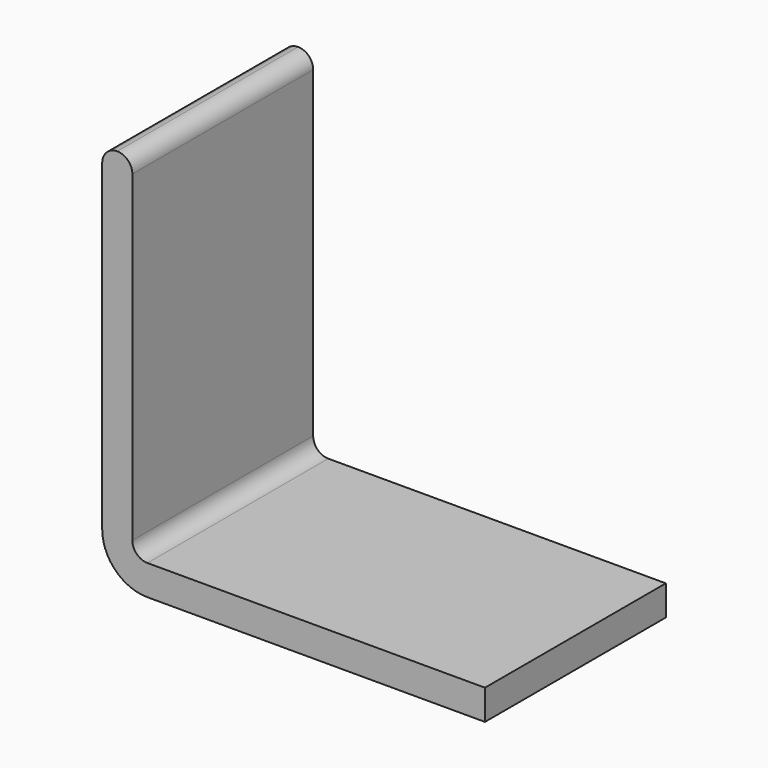
from build123d import *

# Parameters (mm, degrees)
F1_DEPTH = 7.5
F2_R     = 0.99999


# Not quite as in the source:
# - a fillet or chamfer is up to 0.001 mm smaller than in the source, because OpenCascade refuses the exact size


with BuildPart() as f1:
    # F0 (on Front) → F1 (new body, symmetric)
    with BuildSketch(Plane.XZ):
        with BuildLine():
            Line((0, 25.4), (0, 3))
            ThreePointArc((0, 3), (0.8786796564, 0.8786796564), (3, 0))
            Line((3, 0), (25.4, 0))
            Line((25.4, 0), (25.4, 2))
            Line((25.4, 2), (3, 2))
            ThreePointArc((3, 2), (2.2928932188, 2.2928932188), (2, 3))
            Line((2, 3), (2, 25.4))
            Line((2, 25.4), (0, 25.4))
        make_face()
    extrude(amount=F1_DEPTH, both=True)

    # F2 (radius 1 in the source; OpenCascade refuses exactly that, so slightly less here)
    f2_edges = [f1.edges().sort_by_distance(p)[0] for p in [
        (2, 0, 25.4),
        (0, 0, 25.4),
    ]]
    fillet(f2_edges, radius=F2_R)


solid = f1.part
